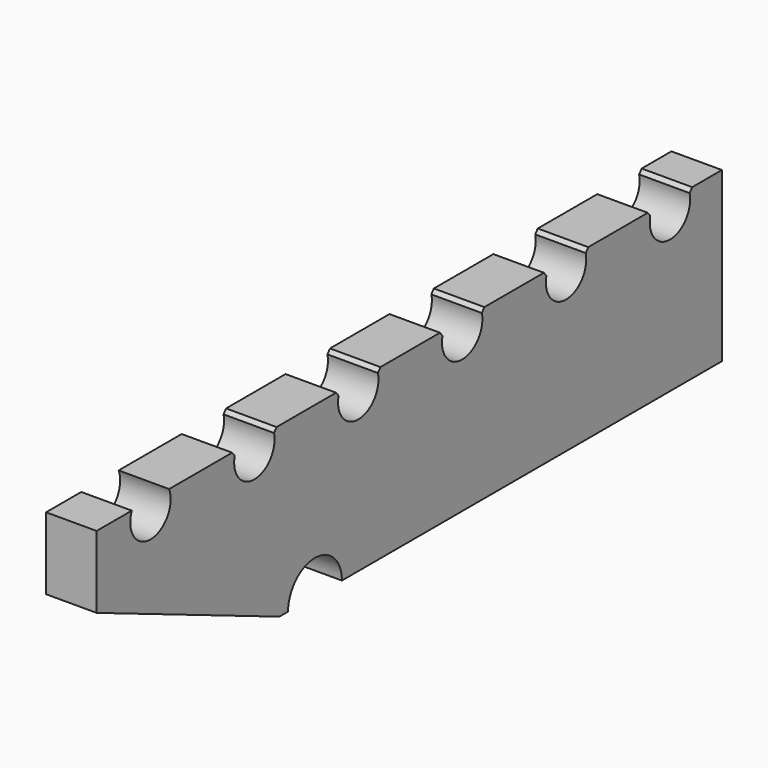
from build123d import *

# Parameters (mm, degrees)
F1_DEPTH    = 21
F2_R        = 10.5
F3_DEPTH    = 25
F4_T1_DEPTH = 30.3938312155
F5_R        = 14
F6_DEPTH    = 25


# Not quite as in the source:
# - a fillet or chamfer that OpenCascade refuses, or shapes differently, is made with other operations: its cross-section is extruded or revolved along the edge and cut away or added


with BuildPart() as f1:
    # F0 (on Right) → F1 (new body)
    with BuildSketch(Plane.YZ):
        Polygon((-134.9917307664, 26.4616465569), (-134.9917307664, -3.5383534431), (-39.9917307664, -43.5383534431), (190.0082692336, -43.5383534431), (190.0082692336, 26.4616465569), align=None)
    extrude(amount=F1_DEPTH)

    # F2 (on face) → F3 (cut)
    with BuildSketch(Plane.YZ.offset(21)):
        with Locations((163.0082692336, 22.4616465569)):
            Circle(F2_R)
        with Locations((109.0082692336, 22.4616465569)):
            Circle(F2_R)
        with Locations((55.0082692336, 22.4616465569)):
            Circle(F2_R)
        with Locations((1.0082692336, 22.4616465569)):
            Circle(F2_R)
        with Locations((-52.9917307664, 22.4616465569)):
            Circle(F2_R)
        with Locations((-106.9917307664, 22.4616465569)):
            Circle(F2_R)
    extrude(amount=-F3_DEPTH, mode=Mode.SUBTRACT)

    # F4: chamfer of 2 on 10 edges, made by hand

    # F4_s2 → F4_t1 (cut)
    with BuildSketch(Plane.YZ.offset(-4.6969156077)):
        with BuildLine():
            Line((-64.5776976071, 26.5242502898), (-63.1732755163, 24.7590076766))
            Line((-63.1732755163, 24.7590076766), (-63.1342989368, 24.7500173343))
            ThreePointArc((-63.1342989368, 24.7500173343), (-62.963845112, 25.6189453198), (-62.6629908996, 26.4464084616))
            Line((-62.6629908996, 26.4464084616), (-62.6999746859, 26.5016465569))
            ThreePointArc((-62.6999746859, 26.5016465569), (-63.6388361465, 26.5016465569), (-64.5776976071, 26.5642502898))
            Line((-64.5776976071, 26.5642502898), (-64.5776976071, 26.5242502898))
        make_face()
        with BuildLine():
            Line((-42.8101860166, 24.7590076766), (-41.4057639258, 26.5242502898))
            Line((-41.4057639258, 26.5242502898), (-41.4057639258, 26.5642502898))
            ThreePointArc((-41.4057639258, 26.5642502898), (-42.3446253864, 26.5016465569), (-43.283486847, 26.5016465569))
            Line((-43.283486847, 26.5016465569), (-43.3204706333, 26.4464084616))
            ThreePointArc((-43.3204706333, 26.4464084616), (-43.0196164209, 25.6189453198), (-42.8491625961, 24.7500173343))
            Line((-42.8491625961, 24.7500173343), (-42.8101860166, 24.7590076766))
        make_face()
        with BuildLine():
            Line((-10.5776976071, 26.5242502898), (-9.1732755163, 24.7590076766))
            Line((-9.1732755163, 24.7590076766), (-9.1342989368, 24.7500173343))
            ThreePointArc((-9.1342989368, 24.7500173343), (-8.963845112, 25.6189453198), (-8.6629908996, 26.4464084616))
            Line((-8.6629908996, 26.4464084616), (-8.6999746859, 26.5016465569))
            ThreePointArc((-8.6999746859, 26.5016465569), (-9.6388361465, 26.5016465569), (-10.5776976071, 26.5642502898))
            Line((-10.5776976071, 26.5642502898), (-10.5776976071, 26.5242502898))
        make_face()
        with BuildLine():
            Line((11.1898139834, 24.7590076766), (12.5942360742, 26.5242502898))
            Line((12.5942360742, 26.5242502898), (12.5942360742, 26.5642502898))
            ThreePointArc((12.5942360742, 26.5642502898), (11.6553746136, 26.5016465569), (10.716513153, 26.5016465569))
            Line((10.716513153, 26.5016465569), (10.6795293667, 26.4464084616))
            ThreePointArc((10.6795293667, 26.4464084616), (10.9803835791, 25.6189453198), (11.1508374039, 24.7500173343))
            Line((11.1508374039, 24.7500173343), (11.1898139834, 24.7590076766))
        make_face()
        with BuildLine():
            Line((43.4223023929, 26.5242502898), (44.8267244837, 24.7590076766))
            Line((44.8267244837, 24.7590076766), (44.8657010632, 24.7500173343))
            ThreePointArc((44.8657010632, 24.7500173343), (45.036154888, 25.6189453198), (45.3370091004, 26.4464084616))
            Line((45.3370091004, 26.4464084616), (45.3000253141, 26.5016465569))
            ThreePointArc((45.3000253141, 26.5016465569), (44.3611638535, 26.5016465569), (43.4223023929, 26.5642502898))
            Line((43.4223023929, 26.5642502898), (43.4223023929, 26.5242502898))
        make_face()
        with BuildLine():
            Line((65.1898139834, 24.7590076766), (66.5942360742, 26.5242502898))
            Line((66.5942360742, 26.5242502898), (66.5942360742, 26.5642502898))
            ThreePointArc((66.5942360742, 26.5642502898), (65.6553746136, 26.5016465569), (64.716513153, 26.5016465569))
            Line((64.716513153, 26.5016465569), (64.6795293667, 26.4464084616))
            ThreePointArc((64.6795293667, 26.4464084616), (64.9803835791, 25.6189453198), (65.1508374039, 24.7500173343))
            Line((65.1508374039, 24.7500173343), (65.1898139834, 24.7590076766))
        make_face()
        with BuildLine():
            Line((97.4223023929, 26.5242502898), (98.8267244837, 24.7590076766))
            Line((98.8267244837, 24.7590076766), (98.8657010632, 24.7500173343))
            ThreePointArc((98.8657010632, 24.7500173343), (99.036154888, 25.6189453198), (99.3370091004, 26.4464084616))
            Line((99.3370091004, 26.4464084616), (99.3000253141, 26.5016465569))
            ThreePointArc((99.3000253141, 26.5016465569), (98.3611638535, 26.5016465569), (97.4223023929, 26.5642502898))
            Line((97.4223023929, 26.5642502898), (97.4223023929, 26.5242502898))
        make_face()
        with BuildLine():
            Line((119.1898139834, 24.7590076766), (120.5942360742, 26.5242502898))
            Line((120.5942360742, 26.5242502898), (120.5942360742, 26.5642502898))
            ThreePointArc((120.5942360742, 26.5642502898), (119.6553746136, 26.5016465569), (118.716513153, 26.5016465569))
            Line((118.716513153, 26.5016465569), (118.6795293667, 26.4464084616))
            ThreePointArc((118.6795293667, 26.4464084616), (118.9803835791, 25.6189453198), (119.1508374039, 24.7500173343))
            Line((119.1508374039, 24.7500173343), (119.1898139834, 24.7590076766))
        make_face()
        with BuildLine():
            Line((151.4223023929, 26.5242502898), (152.8267244837, 24.7590076766))
            Line((152.8267244837, 24.7590076766), (152.8657010632, 24.7500173343))
            ThreePointArc((152.8657010632, 24.7500173343), (153.036154888, 25.6189453198), (153.3370091004, 26.4464084616))
            Line((153.3370091004, 26.4464084616), (153.3000253141, 26.5016465569))
            ThreePointArc((153.3000253141, 26.5016465569), (152.3611638535, 26.5016465569), (151.4223023929, 26.5642502898))
            Line((151.4223023929, 26.5642502898), (151.4223023929, 26.5242502898))
        make_face()
        with BuildLine():
            Line((173.1898139834, 24.7590076766), (174.5942360742, 26.5242502898))
            Line((174.5942360742, 26.5242502898), (174.5942360742, 26.5642502898))
            ThreePointArc((174.5942360742, 26.5642502898), (173.6553746136, 26.5016465569), (172.716513153, 26.5016465569))
            Line((172.716513153, 26.5016465569), (172.6795293667, 26.4464084616))
            ThreePointArc((172.6795293667, 26.4464084616), (172.9803835791, 25.6189453198), (173.1508374039, 24.7500173343))
            Line((173.1508374039, 24.7500173343), (173.1898139834, 24.7590076766))
        make_face()
    extrude(amount=F4_T1_DEPTH, mode=Mode.SUBTRACT)

    # F5 (on face) → F6 (cut)
    with BuildSketch(Plane.YZ.offset(21)):
        with Locations((-21.4917307664, -43.5383534431)):
            Circle(F5_R)
    extrude(amount=-F6_DEPTH, mode=Mode.SUBTRACT)


solid = f1.part
